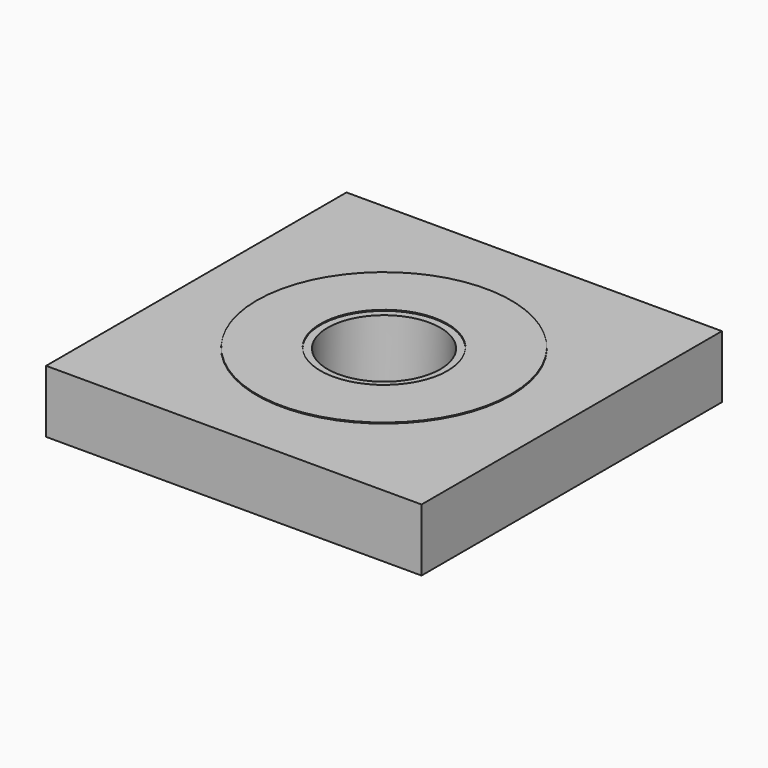
from build123d import *

# Parameters (mm, degrees)
F0_R     = 50.8
F0_R_2   = 25.4
F1_DEPTH = 25.4
F2_W     = 150
F2_H     = 150
F2_R     = 50.8
F3_DEPTH = 25
F4_R     = 25.4
F4_R_2   = 22.5
F5_DEPTH = 25


# Not quite as in the source:
# - the program builds the solid bodies; features that only make, move or delete a surface that nothing else refers to are left out


with BuildPart() as f1:
    # F0 (on Top) → F1 (new body)
    with BuildSketch(Plane.XY):
        Circle(F0_R)
        Circle(F0_R_2, mode=Mode.SUBTRACT)
    extrude(amount=F1_DEPTH)

    # F2 (on Top) → F3 (join)
    with BuildSketch(Plane.XY):
        Rectangle(F2_W, F2_H)
        Circle(F2_R, mode=Mode.SUBTRACT)
    extrude(amount=F3_DEPTH)

    # F4 (on Top) → F5 (join)
    with BuildSketch(Plane.XY):
        Circle(F4_R)
        Circle(F4_R_2, mode=Mode.SUBTRACT)
    extrude(amount=F5_DEPTH)


solid = f1.part
